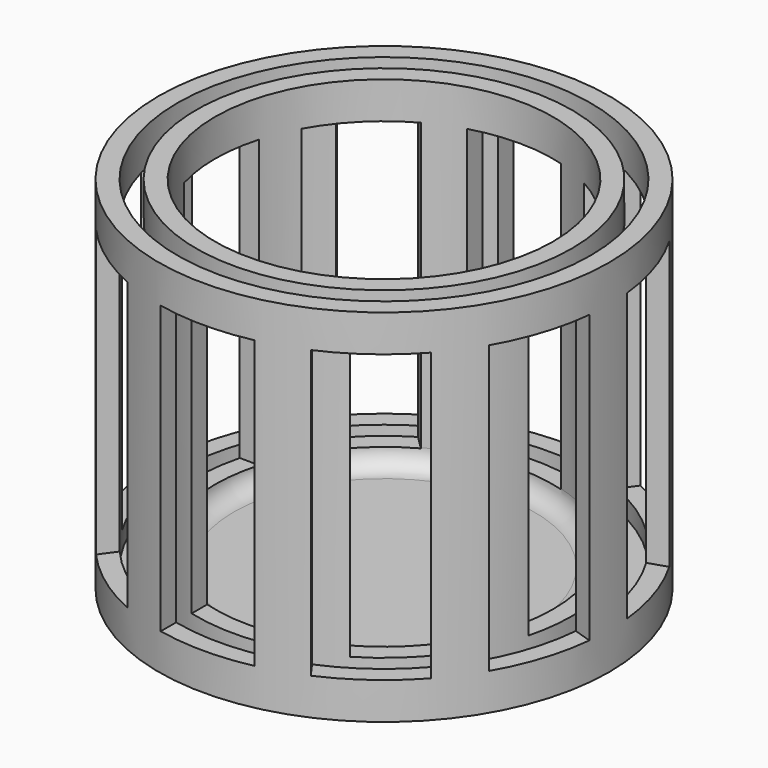
from build123d import *

# Parameters (mm, degrees)
F2_W            = 25
F2_H            = 76.3443418741
F3_REACH        = 140.3344210413
F3_COPIES_COUNT = 8
F5_W            = 25
F5_H            = 76.3443418741
F6_REACH        = 215.3344210413
F6_COPIES_COUNT = 10


# Not quite as in the source:
# - a pattern or mirror of a feature is missing from the dataset's text; its kind, count and spacing are read off the source's solid


with BuildPart() as f1:
    # F0 (on Front) → F1 (revolve)
    with BuildSketch(Plane.XZ):
        with BuildLine():
            Line((0, 5), (0, 0))
            Line((0, 0), (60, 0))
            Line((60, 0), (60, 96))
            Line((60, 96), (55, 96))
            Line((55, 96), (55, 5))
            Line((55, 5), (50, 5))
            Line((50, 5), (50, 96))
            Line((50, 96), (45, 96))
            Line((45, 96), (45, 10))
            ThreePointArc((45, 10), (43.5355339059, 6.4644660941), (40, 5))
            Line((40, 5), (0, 5))
        make_face()
    revolve(axis=Axis((0, 0, 2.5), (0, 0, 1)))

    f3_end = f1.faces().sort_by_distance((-50, 0, 50.5))[0]
    # F2 (on Front) → F3 (cut, up to a face of the model that its end follows)
    with BuildSketch(Plane.XZ):
        with Locations((0, 48)):
            Rectangle(F2_W, F2_H)
    f3_long = extrude(amount=F3_REACH, mode=Mode.PRIVATE)
    f3 = split(f3_long, bisect_by=f3_end, keep=Keep.BOTTOM, mode=Mode.PRIVATE)
    add(f3, mode=Mode.SUBTRACT)

    # F3_copies: F3 ×8 about axis
    f3_copies_axis = Axis((0, 0, 0), (0, 0, 1))
    for i in range(1, F3_COPIES_COUNT):
        add(f3.rotate(f3_copies_axis, i * 360 / F3_COPIES_COUNT), mode=Mode.SUBTRACT)

    f6_end = f1.faces().sort_by_distance((-55, 0, 50.5))[0]
    # F5 (on offset) → F6 (cut, up to a face of the model that its end follows)
    with BuildSketch(Plane.XZ.offset(75)):
        with Locations((0, 48)):
            Rectangle(F5_W, F5_H)
    f6_long = extrude(amount=-F6_REACH, mode=Mode.PRIVATE)
    f6 = split(f6_long, bisect_by=f6_end, keep=Keep.ALL, mode=Mode.PRIVATE).solids().sort_by_distance((0, -75, 48))[0]
    add(f6, mode=Mode.SUBTRACT)

    # F6_copies: F6 ×10 about axis
    f6_copies_axis = Axis((0, 0, 0), (0, 0, 1))
    for i in range(1, F6_COPIES_COUNT):
        add(f6.rotate(f6_copies_axis, i * 360 / F6_COPIES_COUNT), mode=Mode.SUBTRACT)


solid = f1.part
